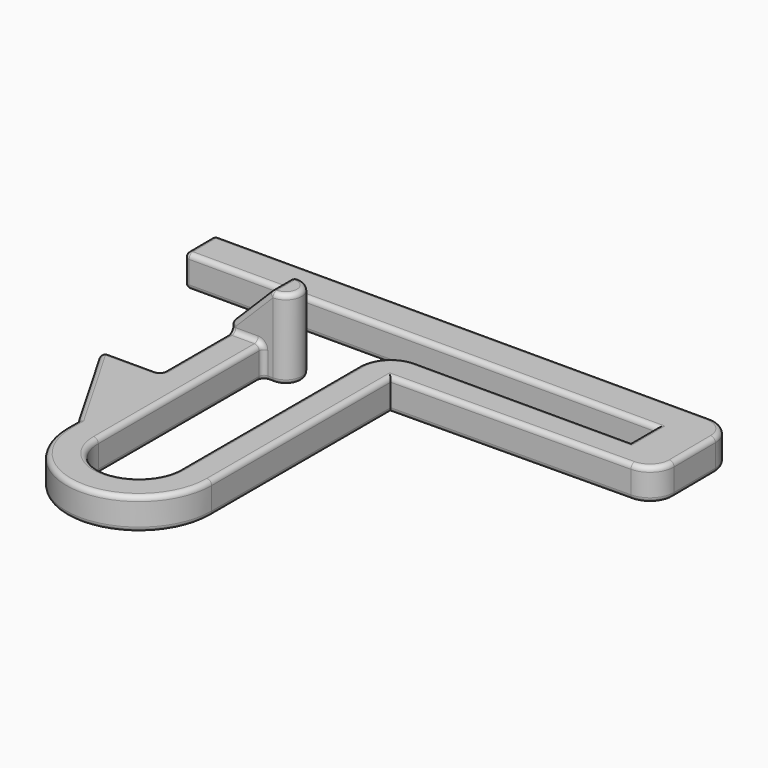
from build123d import *

# Parameters (mm, degrees)
F1_DEPTH = 4
F2_W     = 4
F2_H     = 4
F3_DEPTH = 10
F4_SIZE  = 5
F5_R     = 0.6


with BuildPart() as f1:
    # F0 (on Top) → F1 (new body)
    with BuildSketch(Plane.XY):
        with BuildLine():
            Line((-6.348816124, 12.7998564335), (-68.3719298071, 12.7998564335))
            Line((-68.3719298071, 12.7998564335), (-68.3348054537, 8))
            Line((-68.3348054537, 8), (-9.2984564299, 8))
            Line((-9.2984564299, 8), (-9.2984564299, 4))
            Line((-9.2984564299, 4), (-36.1198379695, 4))
            ThreePointArc((-36.1198379695, 4), (-38.9482650943, 2.8284271247), (-40.1198379695, 0))
            Line((-40.1198379695, 0), (-40.1198379695, -28))
            ThreePointArc((-40.1198379695, -28), (-45.2091471997, -33.0893092302), (-50.2984564299, -28))
            Line((-50.2984564299, -28), (-50.2984564299, 1.7541534589))
            Line((-50.2984564299, 1.7541534589), (-54.2984564299, 1.7541534589))
            Line((-54.2984564299, 1.7541534589), (-54.2984564299, -13.2458465411))
            Line((-54.2984564299, -13.2458465411), (-61.7776213991, -13.2458465411))
            Line((-61.7776213991, -13.2458465411), (-54.2984564299, -26.2001435665))
            Line((-54.2984564299, -26.2001435665), (-54.2984564299, -28))
            ThreePointArc((-54.2984564299, -28), (-45.2091471997, -37.0893092302), (-36.1198379695, -28))
            Line((-36.1198379695, -28), (-36.1198379695, 0))
            Line((-36.1198379695, 0), (-6.2704965664, 0.2773136864))
            ThreePointArc((-6.2704965664, 0.2773136864), (-4.1590662239, 1.1739977225), (-3.2984564299, 3.3003869471))
            Line((-3.2984564299, 3.3003869471), (-3.348905853, 9.8230591544))
            ThreePointArc((-3.348905853, 9.8230591544), (-4.2357151045, 11.929364377), (-6.348816124, 12.7998564335))
        make_face()
    extrude(amount=F1_DEPTH)

    # F2 (on face) → F3 (join)
    with BuildSketch(Plane(origin=(0, 0, 0), x_dir=(1, 0, 0), z_dir=(0, 0, -1))):
        with BuildLine():
            Line((-50.2984564299, -1.7541534589), (-49.0415598922, -1.7541534589))
            ThreePointArc((-49.0415598922, -1.7541534589), (-47.0415598922, 0.2458465411), (-49.0415598922, 2.2458465411))
            Line((-49.0415598922, 2.2458465411), (-50.2984564299, 2.2458465411))
            Line((-50.2984564299, 2.2458465411), (-50.2984564299, -1.7541534589))
        make_face()
        with Locations((-52.2984564299, 0.2458465411)):
            Rectangle(F2_W, F2_H)
    extrude(amount=-F3_DEPTH)

    # F4
    f4_edges = [f1.edges().sort_by_distance(p)[0] for p in [
        (-54.298456, -0.245847, 10),
    ]]
    chamfer(f4_edges, length=F4_SIZE)

    # F5
    f5_edges = [f1.edges().sort_by_distance(p)[0] for p in [
        (-68.353368, 10.399928, 4),
        (-37.360373, 12.799856, 4),
        (-4.235715, 11.929364, 4),
        (-3.323681, 6.561723, 4),
        (-4.159066, 1.173998, 4),
        (-21.195167, 0.138657, 4),
        (-36.119838, -14, 4),
        (-45.209147, -37.089309, 4),
        (-54.298456, -27.100072, 4),
        (-58.038039, -19.722995, 4),
        (-58.038039, -13.245847, 4),
        (-54.298456, -7.745847, 4),
        (-52.298456, -2.245847, 4),
        (-50.298456, -15.122923, 4),
        (-45.209147, -33.089309, 4),
        (-40.119838, -14, 4),
        (-38.948265, 2.828427, 4),
        (-22.709147, 4, 4),
        (-9.298456, 6, 4),
        (-38.816631, 8, 4),
        (-61.777621, -13.245847, 2),
        (-68.334805, 8, 2),
        (-68.37193, 12.799856, 2),
        (-54.298456, 1.754153, 2.5),
        (-51.798456, 1.754153, 7.5),
        (-47.04156, -0.245847, 10),
        (-51.798456, -2.245847, 7.5),
        (-68.353368, 10.399928, 0),
        (-38.816631, 8, 0),
        (-9.298456, 6, 0),
        (-22.709147, 4, 0),
        (-38.948265, 2.828427, 0),
        (-40.119838, -14, 0),
        (-45.209147, -33.089309, 0),
        (-50.298456, -15.122923, 0),
        (-49.670008, -2.245847, 0),
        (-47.04156, -0.245847, 0),
        (-51.670008, 1.754153, 0),
        (-54.298456, -5.745847, 0),
        (-58.038039, -13.245847, 0),
        (-58.038039, -19.722995, 0),
        (-54.298456, -27.100072, 0),
        (-45.209147, -37.089309, 0),
        (-36.119838, -14, 0),
        (-21.195167, 0.138657, 0),
        (-4.159066, 1.173998, 0),
        (-3.323681, 6.561723, 0),
        (-4.235715, 11.929364, 0),
        (-37.360373, 12.799856, 0),
        (-49.298456, -0.245847, 10),
        (-54.298456, -0.245847, 5),
        (-54.298456, -2.245847, 4.5),
        (-54.298456, -13.245847, 2),
        (-50.298456, -2.245847, 2),
    ]]
    fillet(f5_edges, radius=F5_R)


solid = f1.part
